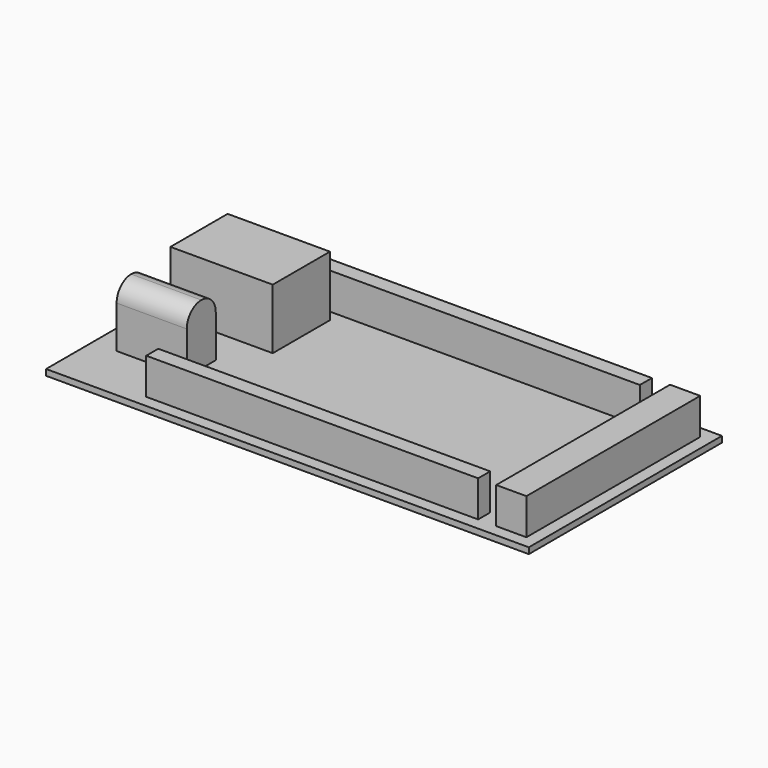
from build123d import *

# Parameters (mm, degrees)
F0_W     = 101.6
F0_H     = 50.8
F1_DEPTH = 1.27
F2_W     = 69.85
F2_H     = 3.175
F2_W_2   = 6.35
F2_H_2   = 45.72
F3_DEPTH = 7.62
F4_W     = 21.532409323
F4_H     = 15.0506472416
F4_W_2   = 14.7617278114
F4_H_2   = 7.62
F5_DEPTH = 12.7
F6_R     = 3.80999


# Not quite as in the source:
# - a fillet or chamfer is up to 0.001 mm smaller than in the source, because OpenCascade refuses the exact size


with BuildPart() as f1:
    # F0 (on Top) → F1 (new body)
    with BuildSketch(Plane.XY):
        Rectangle(F0_W, F0_H)
    extrude(amount=F1_DEPTH)

    # F2 (on face) → F3 (join)
    with BuildSketch(Plane.XY.offset(1.27)):
        with Locations((3.175, 21.2725)):
            Rectangle(F2_W, F2_H)
        with Locations((45.085, 0)):
            Rectangle(F2_W_2, F2_H_2)
        with Locations((3.175, -21.2725)):
            Rectangle(F2_W, F2_H)
    extrude(amount=F3_DEPTH)

    # F4 (on face) → F5 (join)
    with BuildSketch(Plane.XY.offset(1.27)):
        with Locations((-35.9846150789, 9.7787969645)):
            Rectangle(F4_W, F4_H)
        with Locations((-38.3539574899, -9.3564780889)):
            Rectangle(F4_W_2, F4_H_2)
    extrude(amount=F5_DEPTH)

    # F6 (radius 3.81 in the source; OpenCascade refuses exactly that, so slightly less here)
    f6_edges = [f1.edges().sort_by_distance(p)[0] for p in [
        (-38.353957, -13.166478, 13.97),
        (-38.353957, -5.546478, 13.97),
    ]]
    fillet(f6_edges, radius=F6_R)


solid = f1.part
